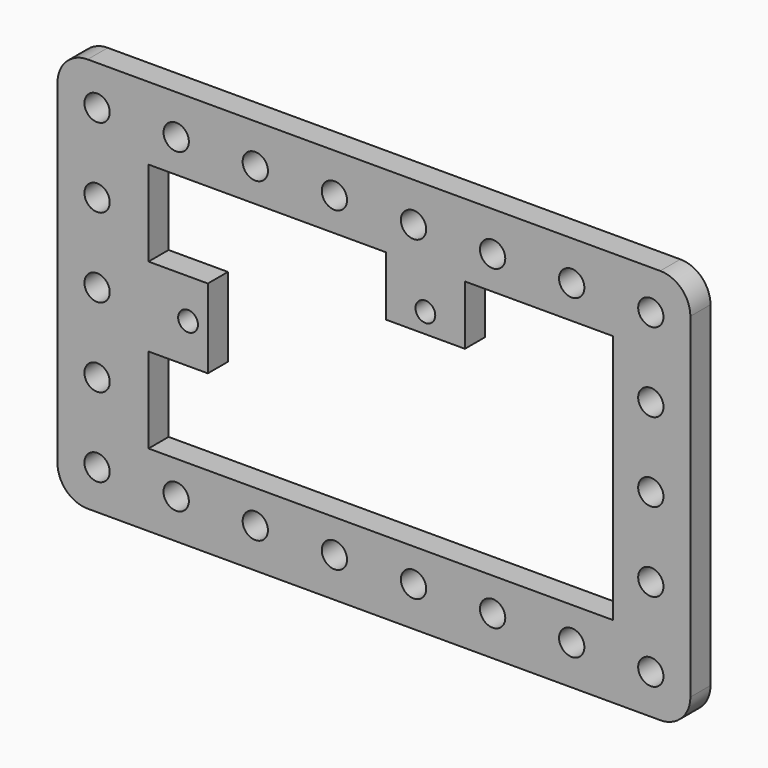
from build123d import *

# Parameters (mm, degrees)
F0_R     = 1.6
F0_R_2   = 1.25
F1_DEPTH = 3.175


# Not quite as in the source:
# - a length typed as a fraction of an inch, garbled in the dataset ("3 / 203.2 mm" for 3/8 in), is restored


with BuildPart() as f1:
    # F0 (on Front) → F1 (new body)
    with BuildSketch(Plane.XZ):
        with BuildLine():
            Line((61.44, 12.45), (-10.94, 12.45))
            ThreePointArc((-10.94, 12.45), (-13.6340768363, 11.3340768363), (-14.75, 8.64))
            Line((-14.75, 8.64), (-14.75, -33.74))
            ThreePointArc((-14.75, -33.74), (-13.6340768363, -36.4340768363), (-10.94, -37.55))
            Line((-10.94, -37.55), (61.44, -37.55))
            ThreePointArc((61.44, -37.55), (64.1340768363, -36.4340768363), (65.25, -33.74))
            Line((65.25, -33.74), (65.25, 8.64))
            ThreePointArc((65.25, 8.64), (64.1340768363, 11.3340768363), (61.44, 12.45))
        make_face()
        with Locations((-9.75, -32.55)):
            Circle(F0_R, mode=Mode.SUBTRACT)
        with Locations((0.25, -32.55)):
            Circle(F0_R, mode=Mode.SUBTRACT)
        with Locations((10.25, -32.55)):
            Circle(F0_R, mode=Mode.SUBTRACT)
        with Locations((20.25, -32.55)):
            Circle(F0_R, mode=Mode.SUBTRACT)
        with Locations((-9.75, -22.55)):
            Circle(F0_R, mode=Mode.SUBTRACT)
        with Locations((30.25, -32.55)):
            Circle(F0_R, mode=Mode.SUBTRACT)
        with Locations((40.25, -32.55)):
            Circle(F0_R, mode=Mode.SUBTRACT)
        with Locations((50.25, -32.55)):
            Circle(F0_R, mode=Mode.SUBTRACT)
        with Locations((60.25, -32.55)):
            Circle(F0_R, mode=Mode.SUBTRACT)
        with Locations((60.25, -22.55)):
            Circle(F0_R, mode=Mode.SUBTRACT)
        with Locations((-9.75, -12.55)):
            Circle(F0_R, mode=Mode.SUBTRACT)
        with Locations((1.75, -12.55)):
            Circle(F0_R_2, mode=Mode.SUBTRACT)
        with Locations((-9.75, -2.55)):
            Circle(F0_R, mode=Mode.SUBTRACT)
        with Locations((-9.75, 7.45)):
            Circle(F0_R, mode=Mode.SUBTRACT)
        with Locations((0.25, 7.45)):
            Circle(F0_R, mode=Mode.SUBTRACT)
        with Locations((10.25, 7.45)):
            Circle(F0_R, mode=Mode.SUBTRACT)
        with Locations((20.25, 7.45)):
            Circle(F0_R, mode=Mode.SUBTRACT)
        Polygon((26.75, -4.25), (36.75, -4.25), (36.75, 3.25), (55.5, 3.25), (55.5, -28.35), (-3.25, -28.35), (-3.25, -17.55), (4.25, -17.55), (4.25, -7.55), (-3.25, -7.55), (-3.25, 3.25), (26.75, 3.25), align=None, mode=Mode.SUBTRACT)
        with Locations((31.75, -1.75)):
            Circle(F0_R_2, mode=Mode.SUBTRACT)
        with Locations((60.25, -12.55)):
            Circle(F0_R, mode=Mode.SUBTRACT)
        with Locations((60.25, -2.55)):
            Circle(F0_R, mode=Mode.SUBTRACT)
        with Locations((30.25, 7.45)):
            Circle(F0_R, mode=Mode.SUBTRACT)
        with Locations((40.25, 7.45)):
            Circle(F0_R, mode=Mode.SUBTRACT)
        with Locations((50.25, 7.45)):
            Circle(F0_R, mode=Mode.SUBTRACT)
        with Locations((60.25, 7.45)):
            Circle(F0_R, mode=Mode.SUBTRACT)
    extrude(amount=F1_DEPTH)


solid = f1.part
